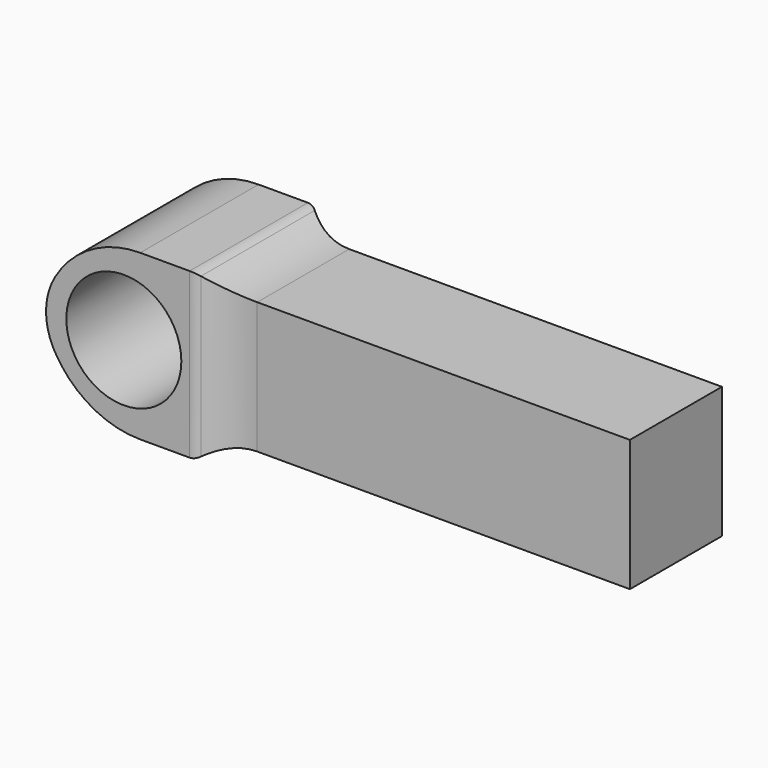
from build123d import *

# Parameters (mm, degrees)
F0_W        = 10
F0_H        = 9
F1_DEPTH    = 5
F3_D        = 7
F4_T1_DEPTH = 39
F5_R        = 1
F6_W        = 7
F6_H        = 8
F7_DEPTH    = 25
F8_R        = 5
F9_R        = 4


# Not quite as in the source:
# - a fillet or chamfer that OpenCascade refuses, or shapes differently, is made with other operations: its cross-section is extruded or revolved along the edge and cut away or added


with BuildPart() as f1:
    # F0 (on Top) → F1 (new body, symmetric)
    with BuildSketch(Plane.XY):
        Rectangle(F0_W, F0_H)
    extrude(amount=F1_DEPTH, both=True)

    # F3 (through all)
    with Locations(Plane(origin=(0, 4.5, 0), x_dir=(-1, 0, 0), z_dir=(0, 1, 0))):
        with Locations((0, 0)):
            Hole(F3_D / 2)

    # F4: fillet of radius 6 on 2 edges, made by hand

    # F4_s2 → F4_t1 (cut)
    with BuildSketch(Plane.XZ.offset(-19.5)):
        with BuildLine():
            ThreePointArc((-5, -1), (-3.2426406871, 3.2426406871), (1, 5))
            Line((1, 5), (-5, 5))
            Line((-5, 5), (-5, -1))
        make_face()
        with BuildLine():
            ThreePointArc((1, -5), (-3.2426406871, -3.2426406871), (-5, 1))
            Line((-5, 1), (-5, -5))
            Line((-5, -5), (1, -5))
        make_face()
    extrude(amount=F4_T1_DEPTH, mode=Mode.SUBTRACT)

    # F5
    f5_edges = [f1.edges().sort_by_distance(p)[0] for p in [
        (5, -4.5, 0),
        (5, 0, -5),
        (5, 4.5, 0),
        (5, 0, 5),
    ]]
    fillet(f5_edges, radius=F5_R)

    # F6 (on face) → F7 (join)
    with BuildSketch(Plane.YZ.offset(5)):
        Rectangle(F6_W, F6_H)
    extrude(amount=F7_DEPTH)

    # F8
    f8_edges = [f1.edges().sort_by_distance(p)[0] for p in [
        (5, 0, 4),
        (5, -3.5, 0),
        (5, 3.5, 0),
        (5, 0, -4),
    ]]
    fillet(f8_edges, radius=F8_R)

    # F9
    f9_edges = [f1.edges().sort_by_distance(p)[0] for p in [
        (-4.91608, 0, 0),
    ]]
    fillet(f9_edges, radius=F9_R)


solid = f1.part
